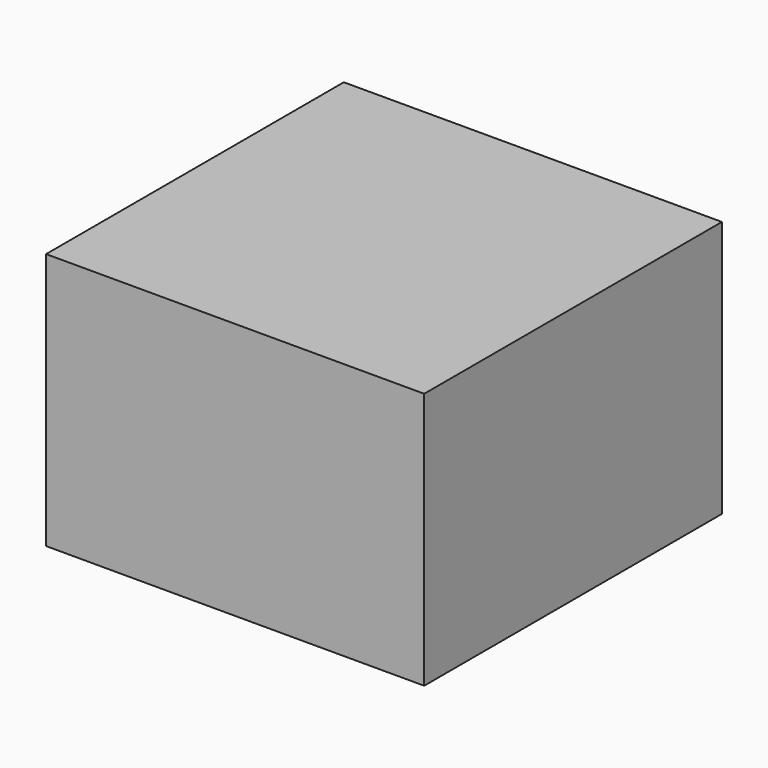
from build123d import *

# Parameters (mm, degrees)
F0_W     = 69.8630958796
F0_H     = 137.5265717506
F3_DEPTH = 94.996


# Not quite as in the source:
# - the program builds the solid bodies; features that only make, move or delete a surface that nothing else refers to are left out


with BuildPart() as f3:
    # F0 (on Top) → F3 (new body)
    with BuildSketch(Plane.XY):
        with Locations((-34.9315479398, 0)):
            Rectangle(F0_W, F0_H)
        with Locations((34.9315479398, 0)):
            Rectangle(F0_W, F0_H)
    extrude(amount=-F3_DEPTH)


solid = f3.part
